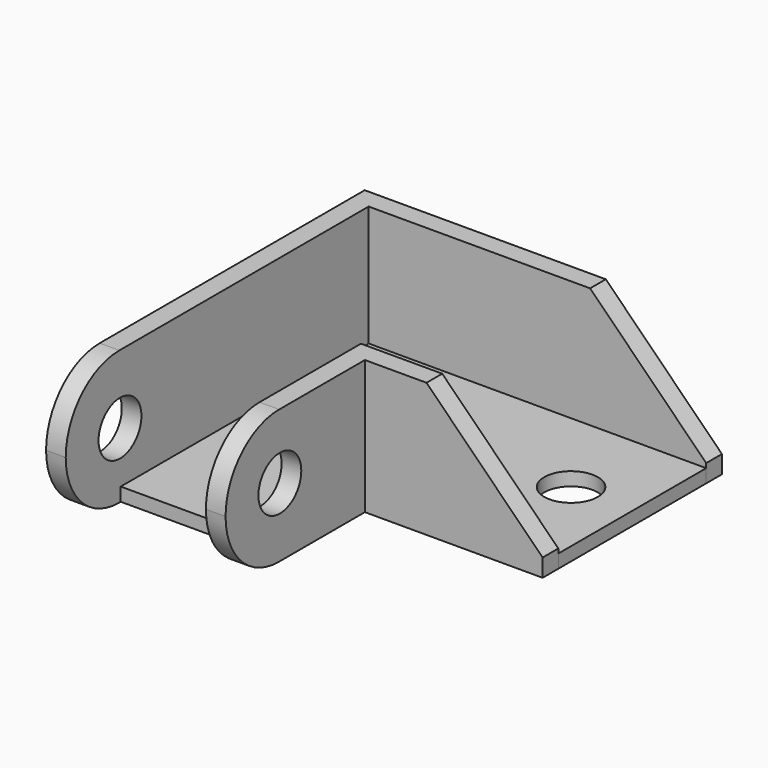
from build123d import *

# Parameters (mm, degrees)
F1_DEPTH   = 15
F0_W       = 19.9
F0_H       = 2.2
F0_W_2     = 2.2
F0_W_3     = 15.7
F0_H_2     = 17.3
F2_DEPTH   = 1.5
F3_R       = 3
F4_DEPTH   = 25
F5_R       = 3
F6_DEPTH   = 25
F7_R       = 3
F8_DEPTH   = 25
F9_R       = 7.49999
F9_2_R     = 7.49999
F10_W      = 15.7
F10_H      = 5.5
F11_DEPTH  = 25
F12_SIZE   = 13
F12_2_SIZE = 13


# Not quite as in the source:
# - a fillet or chamfer is up to 0.001 mm smaller than in the source, because OpenCascade refuses the exact size


with BuildPart() as f1:
    # F0 (on Top) → F1 (new body)
    with BuildSketch(Plane.XY):
        Polygon((0, -2.2), (0, 0), (0, 17.3), (-2.2, 17.3), (-2.2, -2.2), align=None)
        Polygon((-2.2, 17.3), (0, 17.3), (0, 19.5), (0, 40.2), (37.8, 40.2), (37.8, 42.4), (-2.2, 42.4), (-2.2, 19.5), align=None)
    extrude(amount=F1_DEPTH)

    # F7 (on face) → F8 (cut)
    with BuildSketch(Plane(origin=(-2.2, 0, 0), x_dir=(0, -1, 0), z_dir=(-1, 0, 0))):
        with Locations((-5.3973679653, 7.3)):
            Circle(F7_R)
    extrude(amount=-F8_DEPTH, mode=Mode.SUBTRACT)

    # F9 (radius 7.5 in the source; OpenCascade refuses exactly that, so slightly less here)
    f9_edges = [f1.edges().sort_by_distance(p)[0] for p in [
        (-1.1, -2.2, 15),
        (-1.1, -2.2, 0),
    ]]
    fillet(f9_edges, radius=F9_R)

    # F12#2
    f12_2_edges = [f1.edges().sort_by_distance(p)[0] for p in [
        (37.8, 41.3, 15),
    ]]
    chamfer(f12_2_edges, length=F12_2_SIZE)


with BuildPart() as f1b:
    # F0 (on Top) → F1, piece 2 (new body)
    with BuildSketch(Plane.XY):
        Polygon((15.7, 17.3), (15.7, 0), (15.7, -2.2), (17.9, -2.2), (17.9, 17.3), align=None)
        with Locations((27.85, 18.4)):
            Rectangle(F0_W, F0_H)
        with Locations((16.8, 18.4)):
            Rectangle(F0_W_2, F0_H)
    extrude(amount=F1_DEPTH)

    # F5 (on face) → F6 (cut)
    with BuildSketch(Plane.YZ.offset(17.9)):
        with Locations((5.3973679653, 7.7)):
            Circle(F5_R)
    extrude(amount=-F6_DEPTH, mode=Mode.SUBTRACT)

    # F9#2 (radius 7.5 in the source; OpenCascade refuses exactly that, so slightly less here)
    f9_2_edges = [f1b.edges().sort_by_distance(p)[0] for p in [
        (16.8, -2.2, 15),
        (16.8, -2.2, 0),
    ]]
    fillet(f9_2_edges, radius=F9_2_R)

    # F12
    f12_edges = [f1b.edges().sort_by_distance(p)[0] for p in [
        (37.8, 18.4, 15),
    ]]
    chamfer(f12_edges, length=F12_SIZE)


with BuildPart() as f2:
    # F0 (on Top) → F2 (new body)
    with BuildSketch(Plane.XY):
        Polygon((0, 40.2), (0, 19.5), (15.7, 19.5), (17.9, 19.5), (37.8, 19.5), (37.8, 40.2), align=None)
        with Locations((7.85, 8.65)):
            Rectangle(F0_W_3, F0_H_2)
        with Locations((7.85, 18.4)):
            Rectangle(F0_W_3, F0_H)
    extrude(amount=F2_DEPTH)

    # F3 (on face) → F4 (cut)
    with BuildSketch(Plane.XY.offset(1.5)):
        with Locations((30.8023168357, 30.0300842379)):
            Circle(F3_R)
    extrude(amount=-F4_DEPTH, mode=Mode.SUBTRACT)

    # F10 (on face) → F11 (cut)
    with BuildSketch(Plane.XY.offset(1.5)):
        with Locations((7.85, 2.75)):
            Rectangle(F10_W, F10_H)
    extrude(amount=-F11_DEPTH, mode=Mode.SUBTRACT)


solid = Compound([f1.part, f1b.part, f2.part])
